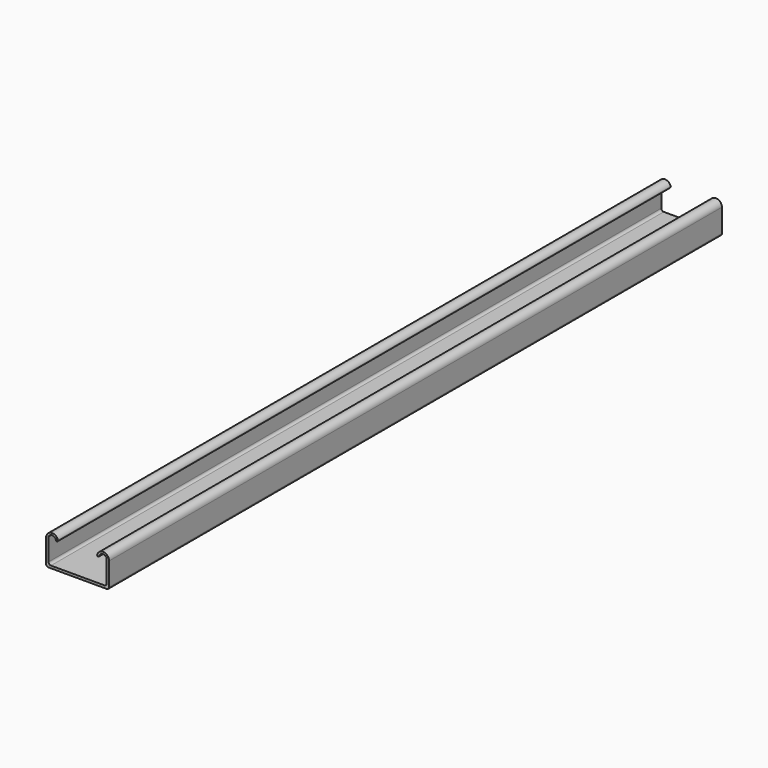
from build123d import *

# Parameters (mm, degrees)
F1_DEPTH    = 250.825
F2_R        = 1.5875
F3_T1_DEPTH = 507.0347591504
F3_T3_DEPTH = 505.1764115156


# Not quite as in the source:
# - a fillet or chamfer that OpenCascade refuses, or shapes differently, is made with other operations: its cross-section is extruded or revolved along the edge and cut away or added


with BuildPart() as f1:
    # F0 (on Front) → F1 (new body, symmetric)
    with BuildSketch(Plane.XZ):
        with BuildLine():
            Line((0, 23.0208111631), (0, 6.3584111631))
            Line((0, 6.3584111631), (41.275, 6.3584111631))
            Line((41.275, 6.3584111631), (41.275, 7.9459111631))
            Line((41.275, 7.9459111631), (41.275, 23.0208111631))
            ThreePointArc((41.275, 23.0208111631), (37.3526007198, 26.9830092528), (33.3510076204, 23.1008085261))
            Line((33.3510076204, 23.1008085261), (34.7028554043, 23.1008085261))
            ThreePointArc((34.7028554043, 23.1008085261), (36.7966084578, 25.5802875082), (39.6875, 24.1057150403))
            Line((39.6875, 24.1057150403), (39.6875, 23.1008085261))
            Line((39.6875, 23.1008085261), (39.6875, 7.9459111631))
            Line((39.6875, 7.9459111631), (1.5875, 7.9459111631))
            Line((1.5875, 7.9459111631), (1.5875, 24.1057150403))
            ThreePointArc((1.5875, 24.1057150403), (4.4783915422, 25.5802875082), (6.5721445957, 23.1008085261))
            Line((6.5721445957, 23.1008085261), (7.9239923796, 23.1008085261))
            ThreePointArc((7.9239923796, 23.1008085261), (3.9223992802, 26.9830092528), (0, 23.0208111631))
        make_face()
    extrude(amount=F1_DEPTH, both=True)

    # F2
    f2_edges = [f1.edges().sort_by_distance(p)[0] for p in [
        (39.6875, 0, 7.945911),
        (1.5875, 0, 7.945911),
        (0, 0, 6.358411),
        (41.275, 0, 6.358411),
    ]]
    fillet(f2_edges, radius=F2_R)

    # F3: fillet of radius 0.8255 on 4 edges, made by hand

    # F3_s2 → F3_t1 (cut)
    with BuildSketch(Plane.XZ.offset(-253.5173795752)):
        with BuildLine():
            ThreePointArc((33.5188726746, 24.1645973059), (33.6466023062, 23.4339961952), (34.309232534, 23.1008085261))
            Line((34.309232534, 23.1008085261), (33.3510076204, 23.1008085261))
            ThreePointArc((33.3510076204, 23.1008085261), (33.3986304583, 23.6384325571), (33.5188726746, 24.1645973059))
        make_face()
        with BuildLine():
            ThreePointArc((7.7561273254, 24.1645973059), (7.6283976938, 23.4339961952), (6.965767466, 23.1008085261))
            Line((6.965767466, 23.1008085261), (7.9239923796, 23.1008085261))
            ThreePointArc((7.9239923796, 23.1008085261), (7.8763695417, 23.6384325571), (7.7561273254, 24.1645973059))
        make_face()
    extrude(amount=F3_T1_DEPTH, mode=Mode.SUBTRACT)

    # F3_s4 → F3_t3 (cut)
    with BuildSketch(Plane.XZ.offset(-252.5882057578)):
        with BuildLine():
            ThreePointArc((33.9975731012, 23.1008085261), (34.4985175119, 23.2701797679), (34.7939002584, 23.7087922999))
            ThreePointArc((34.7939002584, 23.7087922999), (34.7304213855, 23.4074893696), (34.7028554043, 23.1008085261))
            Line((34.7028554043, 23.1008085261), (33.9975731012, 23.1008085261))
        make_face()
        with BuildLine():
            ThreePointArc((7.2774268988, 23.1008085261), (6.7764824881, 23.2701797679), (6.4810997416, 23.7087922999))
            ThreePointArc((6.4810997416, 23.7087922999), (6.5445786145, 23.4074893696), (6.5721445957, 23.1008085261))
            Line((6.5721445957, 23.1008085261), (7.2774268988, 23.1008085261))
        make_face()
    extrude(amount=F3_T3_DEPTH, mode=Mode.SUBTRACT)


solid = f1.part
